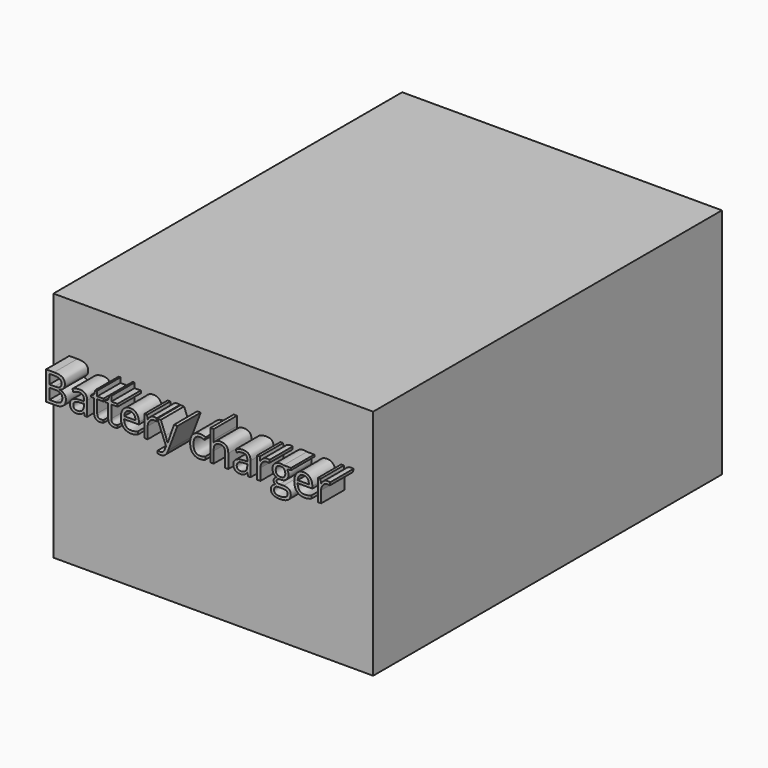
from build123d import *

# Parameters (mm, degrees)
F0_W         = 279.4
F0_H         = 203.2
F1_DEPTH     = 381
F2_TEXT_SIZE = 34.9613953588
F3_DEPTH     = 25.4


# Not quite as in the source:
# - Text() gives the source's letters only with a copy of the font that has no kerning and outlines rounded to 1/6400 em; it was checked with that copy


with BuildPart() as f1:
    # F0 (on Front) → F1 (new body)
    with BuildSketch(Plane.XZ):
        Rectangle(F0_W, F0_H)
    extrude(amount=F1_DEPTH)

    # F2 (on face) → F3 (join)
    with BuildSketch(Plane.XZ.offset(381)):
        with Locations((-129.2304363298, 33.1785020294)):
            Text('Battery charger', F2_TEXT_SIZE, font='Open Sans', text_align=(TextAlign.LEFT, TextAlign.BOTTOM))
    extrude(amount=F3_DEPTH)


solid = f1.part
